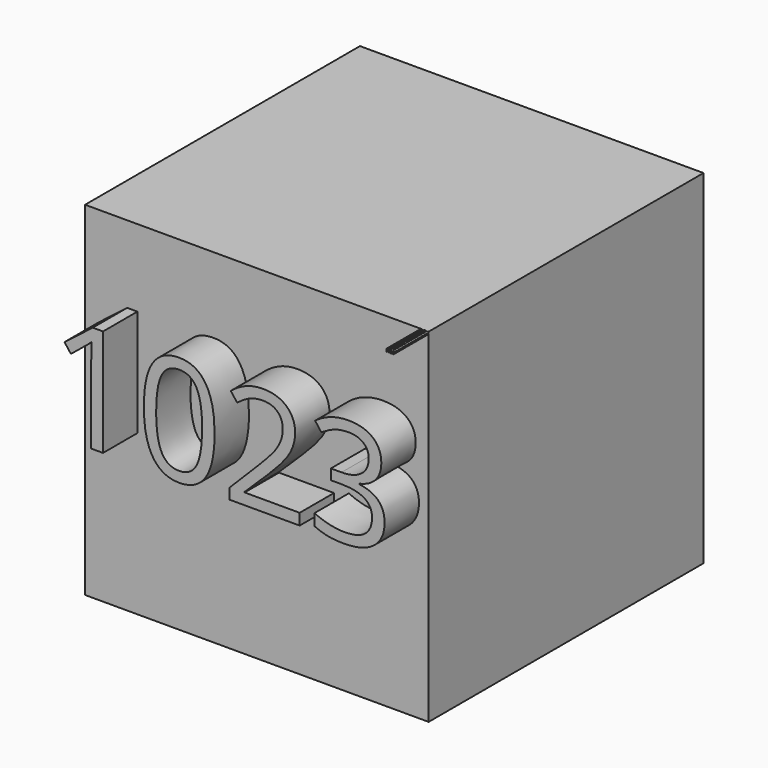
from build123d import *

# Parameters (mm, degrees)
F0_W           = 25.4
F0_H           = 25.4
F1_DEPTH       = 25.4
F2_TEXT_SIZE   = 0.283962975
F2_TEXT_SIZE_2 = 11.0765876261
F3_DEPTH       = 3.175


# Not quite as in the source:
# - Text() gives the source's letters only with a copy of the font that has no kerning and outlines rounded to 1/6400 em; it was checked with that copy


with BuildPart() as f1:
    # F0 (on Front) → F1 (new body)
    with BuildSketch(Plane.XZ):
        Rectangle(F0_W, F0_H)
    extrude(amount=F1_DEPTH)

    # F2 (on face) → F3 (join)
    with BuildSketch(Plane.XZ.offset(25.4)):
        with Locations((12.048837403, 12.495546658)):
            Text('1023', F2_TEXT_SIZE, font='Open Sans', text_align=(TextAlign.LEFT, TextAlign.BOTTOM))
        with Locations((-12.7, -0.9065928766)):
            Text('1023', F2_TEXT_SIZE_2, font='Open Sans', text_align=(TextAlign.LEFT, TextAlign.BOTTOM))
    extrude(amount=F3_DEPTH)


solid = f1.part
